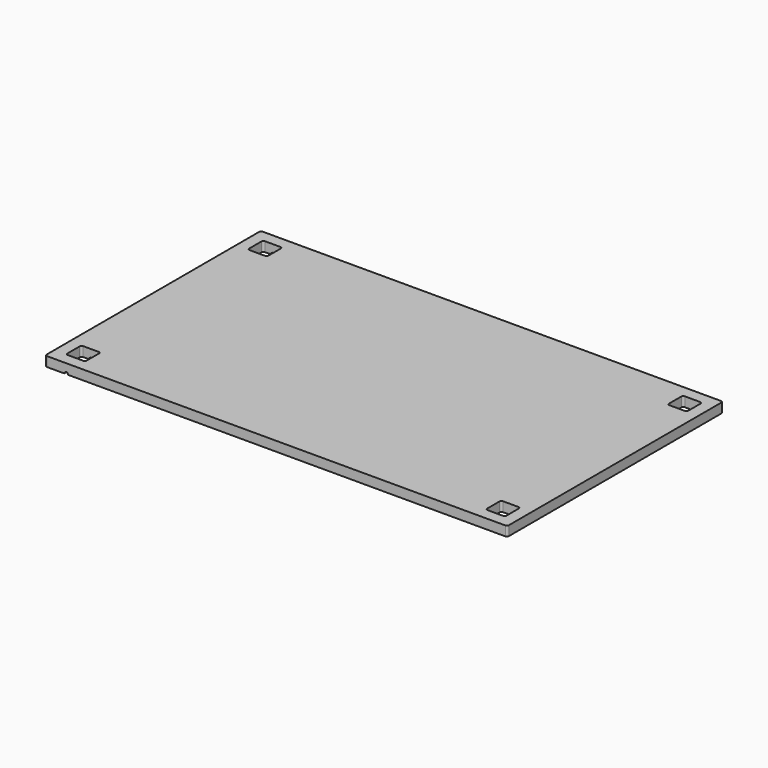
from build123d import *

# Parameters (mm, degrees)
F1_DEPTH = 12.5
F2_W     = 5
F2_H     = 30
F2_H_2   = 540


with BuildPart() as f1:
    # F0 (on Top) → F1 (new body, symmetric)
    with BuildSketch(Plane.XY):
        with BuildLine():
            ThreePointArc((-631.5362024307, 76.3261139393), (-630.0717363367, 72.7905800334), (-626.5362024307, 71.3261139393))
            Line((-626.5362024307, 71.3261139393), (563.4637975693, 71.3261139393))
            ThreePointArc((563.4637975693, 71.3261139393), (566.9993314752, 72.7905800334), (568.4637975693, 76.3261139393))
            Line((568.4637975693, 76.3261139393), (568.4637975693, 766.3261139393))
            ThreePointArc((568.4637975693, 766.3261139393), (566.9993314752, 769.8616478452), (563.4637975693, 771.3261139393))
            Line((563.4637975693, 771.3261139393), (-626.5362024307, 771.3261139393))
            ThreePointArc((-626.5362024307, 771.3261139393), (-630.0717363367, 769.8616478452), (-631.5362024307, 766.3261139393))
            Line((-631.5362024307, 766.3261139393), (-631.5362024307, 76.3261139393))
        make_face()
        with BuildLine():
            ThreePointArc((-601.5362024307, 146.3261139393), (-600.0717363367, 149.8616478452), (-596.5362024307, 151.3261139393))
            Line((-596.5362024307, 151.3261139393), (-556.5362024307, 151.3261139393))
            ThreePointArc((-556.5362024307, 151.3261139393), (-553.0006685248, 149.8616478452), (-551.5362024307, 146.3261139393))
            Line((-551.5362024307, 146.3261139393), (-551.5362024307, 106.3261139393))
            ThreePointArc((-551.5362024307, 106.3261139393), (-553.0006685248, 102.7905800334), (-556.5362024307, 101.3261139393))
            Line((-556.5362024307, 101.3261139393), (-596.5362024307, 101.3261139393))
            ThreePointArc((-596.5362024307, 101.3261139393), (-600.0717363367, 102.7905800334), (-601.5362024307, 106.3261139393))
            Line((-601.5362024307, 106.3261139393), (-601.5362024307, 146.3261139393))
        make_face(mode=Mode.SUBTRACT)
        with BuildLine():
            ThreePointArc((488.4637975693, 146.3261139393), (489.9282636633, 149.8616478452), (493.4637975693, 151.3261139393))
            Line((493.4637975693, 151.3261139393), (533.4637975693, 151.3261139393))
            ThreePointArc((533.4637975693, 151.3261139393), (536.9993314752, 149.8616478452), (538.4637975693, 146.3261139393))
            Line((538.4637975693, 146.3261139393), (538.4637975693, 106.3261139393))
            ThreePointArc((538.4637975693, 106.3261139393), (536.9993314752, 102.7905800334), (533.4637975693, 101.3261139393))
            Line((533.4637975693, 101.3261139393), (493.4637975693, 101.3261139393))
            ThreePointArc((493.4637975693, 101.3261139393), (489.9282636633, 102.7905800334), (488.4637975693, 106.3261139393))
            Line((488.4637975693, 106.3261139393), (488.4637975693, 146.3261139393))
        make_face(mode=Mode.SUBTRACT)
        with BuildLine():
            ThreePointArc((-601.5362024307, 736.3261139393), (-600.0717363367, 739.8616478452), (-596.5362024307, 741.3261139393))
            Line((-596.5362024307, 741.3261139393), (-556.5362024307, 741.3261139393))
            ThreePointArc((-556.5362024307, 741.3261139393), (-553.0006685248, 739.8616478452), (-551.5362024307, 736.3261139393))
            Line((-551.5362024307, 736.3261139393), (-551.5362024307, 696.3261139393))
            ThreePointArc((-551.5362024307, 696.3261139393), (-553.0006685248, 692.7905800334), (-556.5362024307, 691.3261139393))
            Line((-556.5362024307, 691.3261139393), (-596.5362024307, 691.3261139393))
            ThreePointArc((-596.5362024307, 691.3261139393), (-600.0717363367, 692.7905800334), (-601.5362024307, 696.3261139393))
            Line((-601.5362024307, 696.3261139393), (-601.5362024307, 736.3261139393))
        make_face(mode=Mode.SUBTRACT)
        with BuildLine():
            ThreePointArc((488.4637975693, 736.3261139393), (489.9282636633, 739.8616478452), (493.4637975693, 741.3261139393))
            Line((493.4637975693, 741.3261139393), (533.4637975693, 741.3261139393))
            ThreePointArc((533.4637975693, 741.3261139393), (536.9993314752, 739.8616478452), (538.4637975693, 736.3261139393))
            Line((538.4637975693, 736.3261139393), (538.4637975693, 696.3261139393))
            ThreePointArc((538.4637975693, 696.3261139393), (536.9993314752, 692.7905800334), (533.4637975693, 691.3261139393))
            Line((533.4637975693, 691.3261139393), (493.4637975693, 691.3261139393))
            ThreePointArc((493.4637975693, 691.3261139393), (489.9282636633, 692.7905800334), (488.4637975693, 696.3261139393))
            Line((488.4637975693, 696.3261139393), (488.4637975693, 736.3261139393))
        make_face(mode=Mode.SUBTRACT)
    extrude(amount=F1_DEPTH, both=True)

    # F2 (on face) → F3 (revolve, cut)
    with BuildSketch(Plane(origin=(0, 0, -12.5), x_dir=(1, 0, 0), z_dir=(0, 0, -1))):
        with Locations((-574.0362024307, -86.3261139393)):
            Rectangle(F2_W, F2_H)
        with Locations((-574.0362024307, -421.3261139393)):
            Rectangle(F2_W, F2_H_2)
        with Locations((-574.0362024307, -756.3261139393)):
            Rectangle(F2_W, F2_H)
    revolve(axis=Axis((-576.5362024307, 421.3261139393, -12.5), (0, -1, 0)), mode=Mode.SUBTRACT)


solid = f1.part
